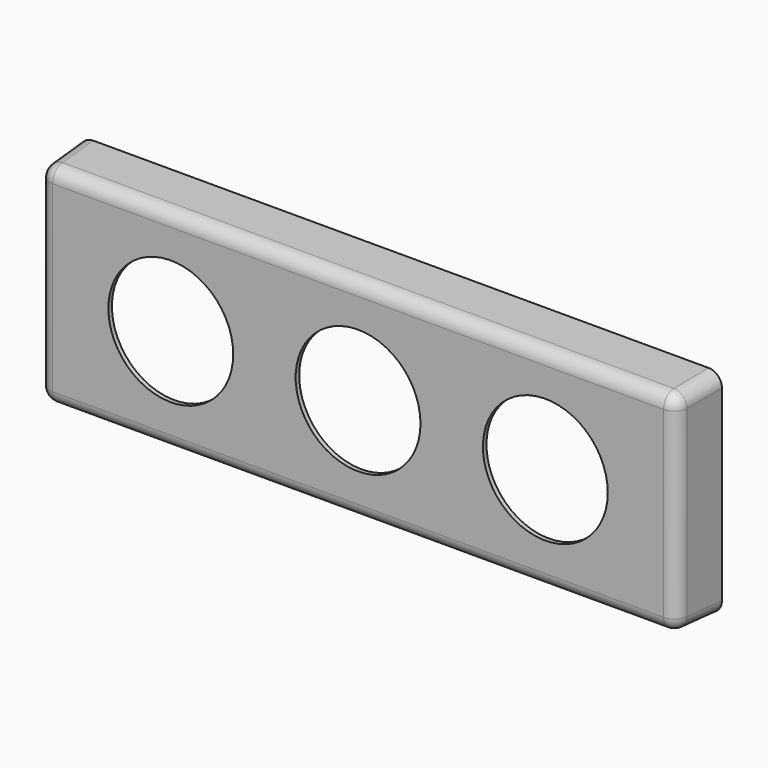
from build123d import *

# Parameters (mm, degrees)
F0_W     = 914.4
F0_H     = 304.8
F1_DEPTH = 76.2
F1_TAPER = 3
F2_R     = 19.05
F3_T     = 6.35
F4_R     = 88.9
F5_DEPTH = 76.2010001


# Not quite as in the source:
# - a shell that OpenCascade refuses in one call is made with other operations: the cavity is built on its own and cut out


with BuildPart() as f1:
    # F0 (on Front) → F1 (new body)
    with BuildSketch(Plane.XZ):
        Rectangle(F0_W, F0_H)
    extrude(amount=F1_DEPTH, taper=F1_TAPER)

    # F2
    f2_edges = [f1.edges().sort_by_distance(p)[0] for p in [
        (455.203264, -38.1, 150.403264),
        (0, -76.2, 148.406527),
        (453.206527, -76.2, 0),
        (455.203264, -38.1, -150.403264),
        (0, -76.2, -148.406527),
        (-455.203264, -38.1, 150.403264),
        (-453.206527, -76.2, 0),
        (-455.203264, -38.1, -150.403264),
    ]]
    fillet(f2_edges, radius=F2_R)

    # F3: shell of thickness 6.35, made by hand


with BuildPart() as f3_core1:
    # F3_t2: copy of F1
    add(f1.part)

    # the walls: a layer under each face that stays
    f3_faces = [f3_core1.faces().sort_by_distance(p)[0] for p in [
        (0, -29.0734999832, 150.8763224299),
        (450.0967392281, -29.2790219143, 145.2967392281),
        (-450.0967392281, -29.2790219142, 145.2967392281),
        (0, -70.9683817678, 143.4419068897),
        (455.6763224299, -29.0734999832, 0),
        (-455.6763224299, -29.0734999832, 0),
        (450.0967392281, -29.2790219142, -145.2967392281),
        (-450.0967392281, -29.2790219142, -145.2967392281),
        (0, -29.0734999832, -150.8763224299),
        (444.4011528131, -70.968381766, 139.6011528105),
        (-448.0884256524, -67.5999269998, 139.5887948951),
        (0, -76.2, 0),
        (448.2419068897, -70.9683817678, 0),
        (-448.2419068897, -70.9683817678, 0),
        (444.388794687, -67.5999269998, -143.2884258011),
        (-448.0884256897, -67.5999270772, -139.5887947556),
        (0, -70.9683817678, -143.4419068897),
    ]]
    thicken(f3_faces, amount=-F3_T, mode=Mode.SUBTRACT)


with BuildPart() as f1_1:
    add(f1.part)

    # what is left inside the walls is the cavity
    f3_cavity = [f3_core1.part.solids().sort_by_distance(p)[0] for p in [
        (29.280349, -0.0635, -87.84086),
    ]]
    add(f3_cavity, mode=Mode.SUBTRACT)

    # F4 (on face) → F5 (cut, through all)
    with BuildSketch(Plane.XZ.offset(76.2)):
        with Locations((266.7, 0)):
            Circle(F4_R)
        Circle(F4_R)
        with Locations((-266.7, 0)):
            Circle(F4_R)
    extrude(amount=-F5_DEPTH, mode=Mode.SUBTRACT)


solid = f1_1.part
